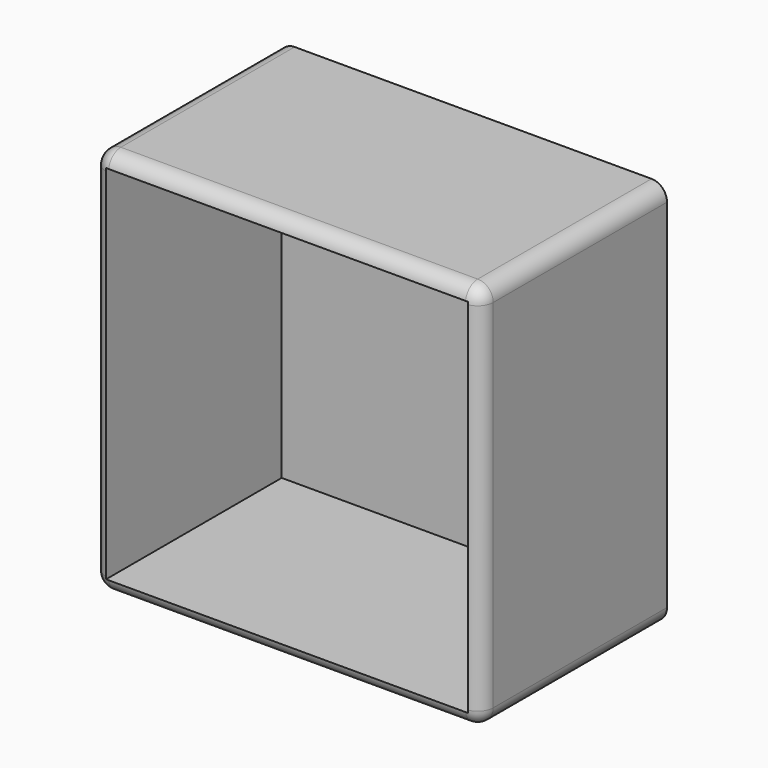
from build123d import *

# Parameters (mm, degrees)
F0_W         = 75
F0_H         = 75
F1_DEPTH     = 45
F2_T         = -2.5
F4_T1_DEPTH  = 49.5
F4_T3_DEPTH  = 69
F4_T5_DEPTH  = 69
F4_S9_W      = 3
F4_S9_H      = 3
F4_T10_DEPTH = 3
F4_S15_W     = 3
F4_S15_H     = 3
F4_T16_DEPTH = 3
F4_S21_W     = 3
F4_S21_H     = 3
F4_T22_DEPTH = 3
F4_S27_W     = 3
F4_S27_H     = 3
F4_T28_DEPTH = 3


# Not quite as in the source:
# - a fillet or chamfer that OpenCascade refuses, or shapes differently, is made with other operations: its cross-section is extruded or revolved along the edge and cut away or added
# - a feature of the source that left no trace in its solid (it failed there, or was rolled back) is left out


with BuildPart() as f1:
    # F0 (on Front) → F1 (new body)
    with BuildSketch(Plane.XZ):
        Rectangle(F0_W, F0_H)
    extrude(amount=F1_DEPTH)

    # F2
    f2_openings = [f1.faces().sort_by_distance(p)[0] for p in [
        (0, -45, 0),
    ]]
    offset(amount=F2_T, openings=f2_openings)

    # F4: fillet of radius 3 on 8 edges, made by hand

    # F4_s2 → F4_t1 (cut)
    with BuildSketch(Plane.XZ.offset(-7.5)):
        with BuildLine():
            ThreePointArc((-34.5, 37.5), (-36.6213203436, 36.6213203436), (-37.5, 34.5))
            Line((-37.5, 34.5), (-37.5, 37.5))
            Line((-37.5, 37.5), (-34.5, 37.5))
        make_face()
        with BuildLine():
            ThreePointArc((-34.5, -37.5), (-36.6213203436, -36.6213203436), (-37.5, -34.5))
            Line((-37.5, -34.5), (-37.5, -37.5))
            Line((-37.5, -37.5), (-34.5, -37.5))
        make_face()
        with BuildLine():
            ThreePointArc((34.5, -37.5), (36.6213203436, -36.6213203436), (37.5, -34.5))
            Line((37.5, -34.5), (37.5, -37.5))
            Line((37.5, -37.5), (34.5, -37.5))
        make_face()
        with BuildLine():
            ThreePointArc((37.5, 34.5), (36.6213203436, 36.6213203436), (34.5, 37.5))
            Line((34.5, 37.5), (37.5, 37.5))
            Line((37.5, 37.5), (37.5, 34.5))
        make_face()
    extrude(amount=F4_T1_DEPTH, mode=Mode.SUBTRACT)

    # F4_s4 → F4_t3 (cut)
    with BuildSketch(Plane.YZ.offset(-34.5)):
        with BuildLine():
            ThreePointArc((-42, -37.5), (-44.1213203436, -36.6213203436), (-45, -34.5))
            Line((-45, -34.5), (-45, -37.5))
            Line((-45, -37.5), (-42, -37.5))
        make_face()
        with BuildLine():
            ThreePointArc((-42, 37.5), (-44.1213203436, 36.6213203436), (-45, 34.5))
            Line((-45, 34.5), (-45, 37.5))
            Line((-45, 37.5), (-42, 37.5))
        make_face()
    extrude(amount=F4_T3_DEPTH, mode=Mode.SUBTRACT)

    # F4_s6 → F4_t5 (cut)
    with BuildSketch(Plane.XY.offset(-34.5)):
        with BuildLine():
            ThreePointArc((37.5, -42), (36.6213203436, -44.1213203436), (34.5, -45))
            Line((34.5, -45), (37.5, -45))
            Line((37.5, -45), (37.5, -42))
        make_face()
        with BuildLine():
            ThreePointArc((-37.5, -42), (-36.6213203436, -44.1213203436), (-34.5, -45))
            Line((-34.5, -45), (-37.5, -45))
            Line((-37.5, -45), (-37.5, -42))
        make_face()
    extrude(amount=F4_T5_DEPTH, mode=Mode.SUBTRACT)


with BuildPart() as f4_tool8:
    # F4_s9 → F4_t10 (new body)
    with BuildSketch(Plane.XY.offset(34.5)):
        with Locations((-36, -43.5)):
            Rectangle(F4_S9_W, F4_S9_H)
    extrude(amount=F4_T10_DEPTH)

    # F4_s11 → F4_t12 (revolve, cut)
    with BuildSketch(Plane(origin=(-34.5, -42, 34.5), x_dir=(0.7071067812, 0.7071067812, 0), z_dir=(0.7071067812, -0.7071067812, 0))):
        with BuildLine():
            ThreePointArc((0, -3), (3, 0), (0, 3))
            Line((0, 3), (0, -3))
        make_face()
    revolve(axis=Axis((-34.5, -42, 34.5), (0, 0, 1)), mode=Mode.SUBTRACT)


with BuildPart() as f1_1:
    add(f1.part)

    # F4_t7: cut F4_tool8
    add(f4_tool8.part, mode=Mode.SUBTRACT)


with BuildPart() as f4_tool14:
    # F4_s15 → F4_t16 (new body)
    with BuildSketch(Plane.XY.offset(-34.5)):
        with Locations((-36, -43.5)):
            Rectangle(F4_S15_W, F4_S15_H)
    extrude(amount=-F4_T16_DEPTH)

    # F4_s17 → F4_t18 (revolve, cut)
    with BuildSketch(Plane(origin=(-34.5, -42, -34.5), x_dir=(0.7071067812, 0.7071067812, 0), z_dir=(-0.7071067812, 0.7071067812, 0))):
        with BuildLine():
            ThreePointArc((0, -3), (3, 0), (0, 3))
            Line((0, 3), (0, -3))
        make_face()
    revolve(axis=Axis((-34.5, -42, -34.5), (0, 0, -1)), mode=Mode.SUBTRACT)


with BuildPart() as f1_2:
    add(f1_1.part)

    # F4_t13: cut F4_tool14
    add(f4_tool14.part, mode=Mode.SUBTRACT)


with BuildPart() as f4_tool20:
    # F4_s21 → F4_t22 (new body)
    with BuildSketch(Plane.XY.offset(-34.5)):
        with Locations((36, -43.5)):
            Rectangle(F4_S21_W, F4_S21_H)
    extrude(amount=-F4_T22_DEPTH)

    # F4_s23 → F4_t24 (revolve, cut)
    with BuildSketch(Plane(origin=(34.5, -42, -34.5), x_dir=(-0.7071067812, 0.7071067812, 0), z_dir=(-0.7071067812, -0.7071067812, 0))):
        with BuildLine():
            ThreePointArc((0, -3), (3, 0), (0, 3))
            Line((0, 3), (0, -3))
        make_face()
    revolve(axis=Axis((34.5, -42, -34.5), (0, 0, -1)), mode=Mode.SUBTRACT)


with BuildPart() as f1_3:
    add(f1_2.part)

    # F4_t19: cut F4_tool20
    add(f4_tool20.part, mode=Mode.SUBTRACT)


with BuildPart() as f4_tool26:
    # F4_s27 → F4_t28 (new body)
    with BuildSketch(Plane.YZ.offset(34.5)):
        with Locations((-43.5, 36)):
            Rectangle(F4_S27_W, F4_S27_H)
    extrude(amount=F4_T28_DEPTH)

    # F4_s29 → F4_t30 (revolve, cut)
    with BuildSketch(Plane(origin=(34.5, -42, 34.5), x_dir=(0, 0.7071067812, -0.7071067812), z_dir=(0, -0.7071067812, -0.7071067812))):
        with BuildLine():
            ThreePointArc((0, -3), (3, 0), (0, 3))
            Line((0, 3), (0, -3))
        make_face()
    revolve(axis=Axis((34.5, -42, 34.5), (1, 0, 0)), mode=Mode.SUBTRACT)


with BuildPart() as f1_4:
    add(f1_3.part)

    # F4_t25: cut F4_tool26
    add(f4_tool26.part, mode=Mode.SUBTRACT)


solid = f1_4.part
